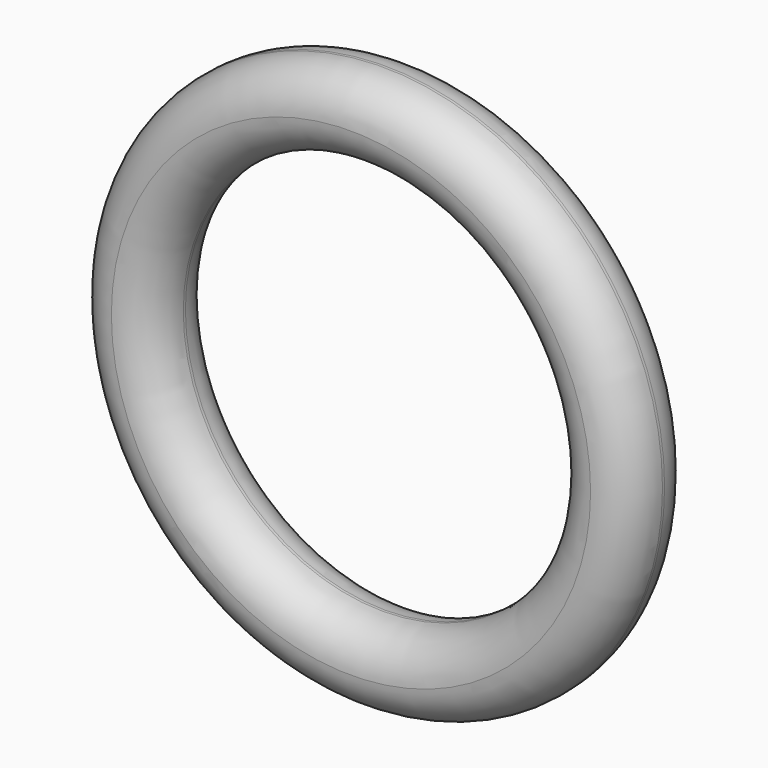
from build123d import *

# Parameters (mm, degrees)
F0_R     = 10.5
F0_R_2   = 7.5
F1_DEPTH = 1.55
F2_R     = 1.49999


# Not quite as in the source:
# - a fillet or chamfer is up to 0.001 mm smaller than in the source, because OpenCascade refuses the exact size


with BuildPart() as f1:
    # F0 (on Front) → F1 (new body, symmetric)
    with BuildSketch(Plane.XZ):
        Circle(F0_R)
        Circle(F0_R_2, mode=Mode.SUBTRACT)
    extrude(amount=F1_DEPTH, both=True)

    # F2 (radius 1.5 in the source; OpenCascade refuses exactly that, so slightly less here)
    f2_edges = [f1.edges().sort_by_distance(p)[0] for p in [
        (-10.5, -1.55, 0),
        (-10.5, 1.55, 0),
        (-7.5, 1.55, 0),
        (-7.5, -1.55, 0),
    ]]
    fillet(f2_edges, radius=F2_R)


solid = f1.part
